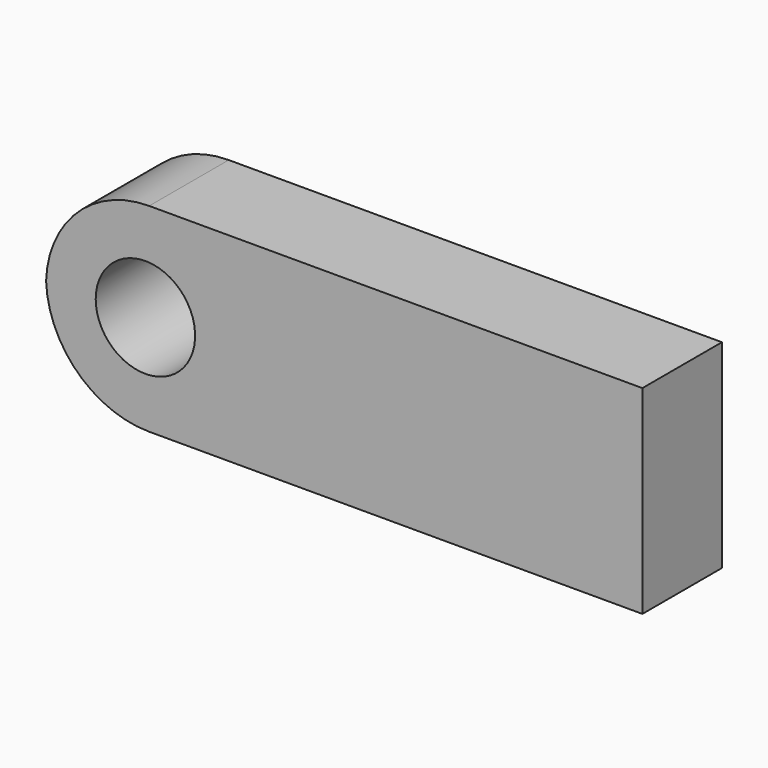
from build123d import *

# Parameters (mm, degrees)
F1_DEPTH    = 10
F2_T1_DEPTH = 61.905591591


# Not quite as in the source:
# - a fillet or chamfer that OpenCascade refuses, or shapes differently, is made with other operations: its cross-section is extruded or revolved along the edge and cut away or added


with BuildPart() as f1:
    # F0 (on Front) → F1 (new body)
    with BuildSketch(Plane.XZ):
        Polygon((-34.8533578217, 10), (-34.8533578217, 0), (25.1466421783, 0), (25.1466421783, 20), (-34.8533578217, 20), align=None)
        with BuildLine():
            ThreePointArc((-19.8533578217, 10), (-24.8533578217, 5), (-29.8533578217, 10))
            ThreePointArc((-29.8533578217, 10), (-24.8533578217, 15), (-19.8533578217, 10))
        make_face(mode=Mode.SUBTRACT)
    extrude(amount=F1_DEPTH)

    # F2: fillet of radius 10.3811183182 on 2 edges, made by hand

    # F2_s2 → F2_t1 (cut)
    with BuildSketch(Plane.XZ.offset(-25.9527957955)):
        with BuildLine():
            ThreePointArc((-24.4722395035, 20), (-31.8127986626, 16.9594408409), (-34.8533578217, 9.6188816818))
            Line((-34.8533578217, 9.6188816818), (-34.8533578217, 20))
            Line((-34.8533578217, 20), (-24.4722395035, 20))
        make_face()
        with BuildLine():
            ThreePointArc((-24.4722395035, 0), (-31.8127986626, 3.0405591591), (-34.8533578217, 10.3811183182))
            Line((-34.8533578217, 10.3811183182), (-34.8533578217, 0))
            Line((-34.8533578217, 0), (-24.4722395035, 0))
        make_face()
    extrude(amount=F2_T1_DEPTH, mode=Mode.SUBTRACT)


solid = f1.part
